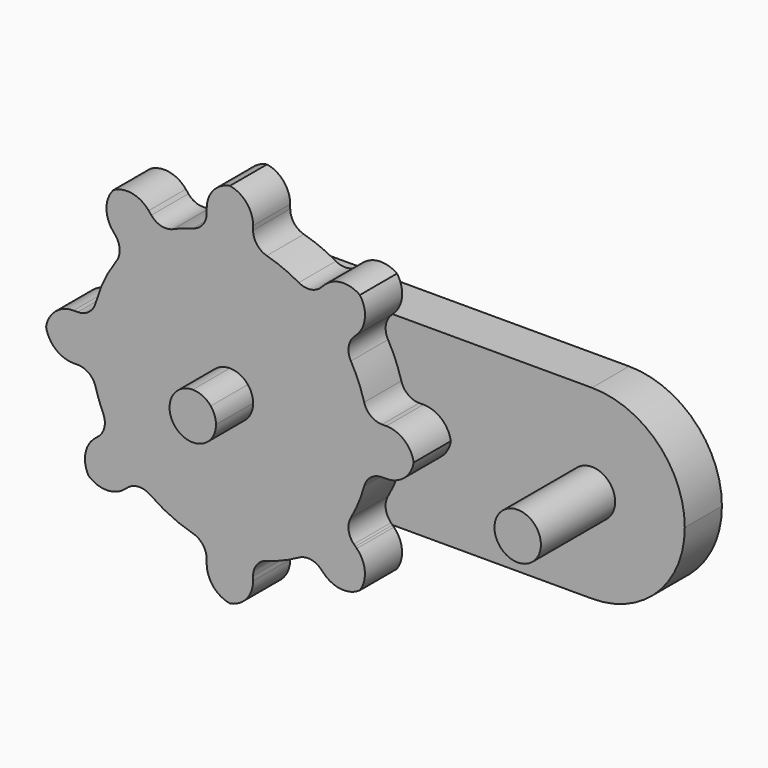
from build123d import *

# Parameters (mm, degrees)
F1_DEPTH    = 12.7
F3_DEPTH    = 25.4
F4_DEPTH    = 12.7
F5_T1_DEPTH = 50.8
F5_T3_DEPTH = 50.8226057065
F5_T5_DEPTH = 50.8231682345
F5_T7_DEPTH = 51.3109317266
F2_R        = 6.35
F6_DEPTH    = 25.4
F7_R        = 5.08


# Not quite as in the source:
# - a fillet or chamfer that OpenCascade refuses, or shapes differently, is made with other operations: its cross-section is extruded or revolved along the edge and cut away or added
# - a feature names something its author has since deleted; it is built from what else it names


with BuildPart() as f1:
    # F0 (on Front) → F1 (new body)
    with BuildSketch(Plane.XZ):
        with BuildLine():
            Line((50.8, 25.4), (0, 25.4))
            Line((0, 25.4), (-50.8, 25.4))
            ThreePointArc((-50.8, 25.4), (-32.8394877579, 17.9605122421), (-25.4, 0))
            ThreePointArc((-25.4, 0), (-32.8394877579, -17.9605122421), (-50.8, -25.4))
            Line((-50.8, -25.4), (50.8, -25.4))
            ThreePointArc((50.8, -25.4), (25.4, 0), (50.8, 25.4))
        make_face()
        with BuildLine():
            ThreePointArc((76.2, 0), (68.7605122421, 17.9605122421), (50.8, 25.4))
            Line((50.8, 25.4), (50.8, 0))
            Line((50.8, 0), (50.8, -25.4))
            ThreePointArc((50.8, -25.4), (68.7605122421, -17.9605122421), (76.2, 0))
        make_face()
        with BuildLine():
            Line((50.8, 0), (50.8, 25.4))
            ThreePointArc((50.8, 25.4), (25.4, 0), (50.8, -25.4))
            Line((50.8, -25.4), (50.8, 0))
        make_face()
        with BuildLine():
            ThreePointArc((-25.4, 0), (-32.8394877579, 17.9605122421), (-50.8, 25.4))
            Line((-50.8, 25.4), (-50.8, -25.4))
            ThreePointArc((-50.8, -25.4), (-32.8394877579, -17.9605122421), (-25.4, 0))
        make_face()
        with BuildLine():
            Line((-50.8, -25.4), (-50.8, 25.4))
            ThreePointArc((-50.8, 25.4), (-76.2, 0), (-50.8, -25.4))
        make_face()
    extrude(amount=F1_DEPTH)

    # F2 (on face) → F3 (join)
    with BuildSketch(Plane.XZ.offset(12.7)):
        with BuildLine():
            Line((-38.1, 0), (-38.1, 6.35))
            ThreePointArc((-38.1, 6.35), (-40.5300397853, 5.8666350357), (-42.5901280449, 4.4901280762))
            ThreePointArc((-42.5901280449, 4.4901280762), (-43.3184117467, 3.6181043161), (-43.8796412291, 2.6302561211))
            ThreePointArc((-43.8796412291, 2.6302561211), (-44.3057723857, 1.3456927946), (-44.45, 0))
            Line((-44.45, 0), (-38.1, 0))
        make_face()
        with BuildLine():
            ThreePointArc((-31.75, 0), (-32.1210860167, 2.1389454365), (-33.1909724663, 4.0278963086))
            ThreePointArc((-33.1909724663, 4.0278963086), (-35.384732201, 5.7401934445), (-38.1, 6.35))
            Line((-38.1, 6.35), (-38.1, 0))
            Line((-38.1, 0), (-31.75, 0))
        make_face()
        with BuildLine():
            ThreePointArc((-34.0440592308, -4.8858821595), (-32.3520558508, -2.6988216054), (-31.75, 0))
            Line((-31.75, 0), (-38.1, 0))
            Line((-38.1, 0), (-38.1, -6.35))
            ThreePointArc((-38.1, -6.35), (-35.9439447726, -5.9727653442), (-34.0440592308, -4.8858821595))
        make_face()
        with BuildLine():
            ThreePointArc((-42.1396767001, -4.8993379307), (-40.2461248962, -5.9763406805), (-38.1, -6.35))
            Line((-38.1, -6.35), (-38.1, 0))
            Line((-38.1, 0), (-44.45, 0))
            ThreePointArc((-44.45, 0), (-44.0789139833, -2.1389454365), (-43.0090275337, -4.0278963086))
            Line((-43.0090275337, -4.0278963086), (-42.1396767001, -4.8993379307))
        make_face()
    extrude(amount=F3_DEPTH)

    # F2 (on face) → F6 (join)
    with BuildSketch(Plane.XZ.offset(12.7)):
        with Locations((50.8, 0)):
            Circle(F2_R)
    extrude(amount=F6_DEPTH)


with BuildPart() as f4:
    # F2 (on face) → F4 (new body)
    with BuildSketch(Plane.XZ.offset(12.7)):
        with BuildLine():
            ThreePointArc((-44.45, 37.5671066227), (-38.1, 38.1), (-31.75, 37.5671066227))
            Line((-31.75, 37.5671066227), (-31.75, 50.4015624758))
            Line((-31.75, 50.4015624758), (-44.45, 50.4015624758))
            Line((-44.45, 50.4015624758), (-44.45, 37.5671066227))
        make_face()
        with BuildLine():
            Line((-21.6802561211, 25.4), (-16.0261722181, 31.054083903))
            ThreePointArc((-16.0261722181, 31.054083903), (-23.5197612269, 35.1998101887), (-31.75, 37.5671066227))
            Line((-31.75, 37.5671066227), (-31.75, 25.4))
            Line((-31.75, 25.4), (-21.6802561211, 25.4))
        make_face()
        Polygon((-40.7302561211, 6.35), (-37.6355270345, 9.4447290866), (-44.45, 17.7499169198), (-44.45, 6.35), align=None)
        Polygon((-44.45, 17.7499169198), (-44.45, 25.4), (-50.7269542822, 25.4), align=None)
        Polygon((-44.45, 2.6302561211), (-44.45, 6.35), (-51.5241743618, 6.35), (-46.6414025016, 0.3990867524), (-44.45, 2.1694751581), align=None)
        with BuildLine():
            Line((-75.3934442484, 6.35), (-51.5241743618, 6.35))
            Line((-51.5241743618, 6.35), (-64.0796310794, 21.6520529834))
            ThreePointArc((-64.0796310794, 21.6520529834), (-71.2237769542, 15.1006402158), (-75.3934442484, 6.35))
        make_face()
        Polygon((-35.0962770958, 6.35), (-31.75, 6.35), (-31.75, 15.3302561211), (-37.6355270345, 9.4447290866), align=None)
        with BuildLine():
            ThreePointArc((-62.9493278972, -28.8811513458), (-54.2929296323, -34.4876648952), (-44.45, -37.5671066227))
            Line((-44.45, -37.5671066227), (-44.45, -25.4))
            Line((-44.45, -25.4), (-50.8, -25.4))
            ThreePointArc((-50.8, -25.4), (-54.2464658379, -25.1650923548), (-57.6291835519, -24.4647144274))
            Line((-57.6291835519, -24.4647144274), (-62.9493278972, -28.8811513458))
        make_face()
        with BuildLine():
            Line((-46.6414025016, 0.3990867524), (-51.5241743618, 6.35))
            Line((-51.5241743618, 6.35), (-75.3934442484, 6.35))
            ThreePointArc((-75.3934442484, 6.35), (-75.9975542735, 3.2005091207), (-76.2, 1.847e-07))
            ThreePointArc((-76.2, 1.847e-07), (-75.9975542968, -3.2005089374), (-75.3934442484, -6.35))
            Line((-75.3934442484, -6.35), (-54.9954820613, -6.35))
            Line((-54.9954820613, -6.35), (-46.6414025016, 0.3990867524))
        make_face()
        with BuildLine():
            ThreePointArc((-31.75, -37.5671066227), (-23.5268945025, -35.2027640415), (-16.0387597828, -31.0630275421))
            Line((-16.0387597828, -31.0630275421), (-21.6882004226, -25.4))
            Line((-21.6882004226, -25.4), (-31.75, -25.4))
            Line((-31.75, -25.4), (-31.75, -37.5671066227))
        make_face()
        with BuildLine():
            Line((-3.7630761576, -25.4), (-7.0639290773, -22.0991470804))
            ThreePointArc((-7.0639290773, -22.0991470804), (-8.337137476, -23.786172756), (-9.7019366858, -25.4))
            Line((-9.7019366858, -25.4), (-3.7630761576, -25.4))
        make_face()
        with BuildLine():
            ThreePointArc((-16.0261722181, 31.054083903), (-12.7061993018, 28.4036069206), (-9.7019366858, 25.4))
            Line((-9.7019366858, 25.4), (-3.7197438789, 25.4))
            Line((-3.7197438789, 25.4), (2.0294146696, 31.1491585485))
            Line((2.0294146696, 31.1491585485), (-6.9508414515, 40.1294146696))
            Line((-6.9508414515, 40.1294146696), (-16.0261722181, 31.054083903))
        make_face()
        with BuildLine():
            Line((-21.6802561211, 25.4), (-9.7019366858, 25.4))
            ThreePointArc((-9.7019366858, 25.4), (-12.7061993018, 28.4036069206), (-16.0261722181, 31.054083903))
            Line((-16.0261722181, 31.054083903), (-21.6802561211, 25.4))
        make_face()
        Polygon((-44.45, -13.5242156334), (-38.479730006, -8.568086795), (-40.6924951019, -6.35), (-44.45, -6.35), align=None)
        with BuildLine():
            ThreePointArc((-75.6671066227, -6.35), (-73.9071383493, -13.0176358542), (-70.974125446, -19.2588129479))
            Line((-70.974125446, -19.2588129479), (-69.0293061757, -17.6876339953))
            ThreePointArc((-69.0293061757, -17.6876339953), (-72.9490964742, -12.4329210315), (-75.3934442484, -6.35))
            Line((-75.3934442484, -6.35), (-75.6671066227, -6.35))
        make_face()
        with BuildLine():
            Line((-57.6291835519, -24.4647144274), (-44.45, -13.5242156334))
            Line((-44.45, -13.5242156334), (-44.45, -6.35))
            Line((-44.45, -6.35), (-54.9954820613, -6.35))
            Line((-54.9954820613, -6.35), (-69.0293061757, -17.6876339953))
            ThreePointArc((-69.0293061757, -17.6876339953), (-63.7793752413, -21.8333647967), (-57.6291835519, -24.4647144274))
        make_face()
        with BuildLine():
            ThreePointArc((-9.7019366858, -25.4), (-8.337137476, -23.786172756), (-7.0639290773, -22.0991470804))
            Line((-7.0639290773, -22.0991470804), (-22.8130761576, -6.35))
            Line((-22.8130761576, -6.35), (-31.75, -6.35))
            Line((-31.75, -6.35), (-31.75, -15.3140017988))
            Line((-31.75, -15.3140017988), (-21.6882004226, -25.4))
            Line((-21.6882004226, -25.4), (-9.7019366858, -25.4))
        make_face()
        with BuildLine():
            ThreePointArc((-76.2, 1.847e-07), (-76.0665429105, 3.1861606087), (-75.6671066227, 6.35))
            Line((-75.6671066227, 6.35), (-88.5015624758, 6.35))
            Line((-88.5015624758, 6.35), (-88.5015624758, -6.35))
            Line((-88.5015624758, -6.35), (-75.6671066227, -6.35))
            ThreePointArc((-75.6671066227, -6.35), (-76.066542926, -3.1861604246), (-76.2, 1.847e-07))
        make_face()
        with BuildLine():
            ThreePointArc((-0.5328933773, 6.35), (-0.1334570818, 3.1861605167), (0, 0))
            ThreePointArc((0, 0), (-0.1334570818, -3.1861605167), (-0.5328933773, -6.35))
            Line((-0.5328933773, -6.35), (12.3015624758, -6.35))
            Line((12.3015624758, -6.35), (12.3015624758, 6.35))
            Line((12.3015624758, 6.35), (-0.5328933773, 6.35))
        make_face()
        with BuildLine():
            ThreePointArc((-0.5328933773, -6.35), (-0.1334570818, -3.1861605167), (0, 0))
            ThreePointArc((0, 0), (-0.1334570818, 3.1861605167), (-0.5328933773, 6.35))
            Line((-0.5328933773, 6.35), (-22.7697438789, 6.35))
            Line((-22.7697438789, 6.35), (-29.1414100183, -0.0216661394))
            Line((-29.1414100183, -0.0216661394), (-22.8130761576, -6.35))
            Line((-22.8130761576, -6.35), (-0.5328933773, -6.35))
        make_face()
        Polygon((-54.9954820613, -6.35), (-44.45, -6.35), (-44.45, -2.2717007737), (-46.6414025016, 0.3990867524), align=None)
        Polygon((-31.75, -25.4), (-31.75, -15.3140017988), (-38.479730006, -8.568086795), (-44.45, -13.5242156334), (-44.45, -25.4), align=None)
        Polygon((-29.1414100183, -0.0216661394), (-22.7697438789, 6.35), (-31.75, 6.35), (-31.75, 2.5869238424), align=None)
        with BuildLine():
            Line((-44.45, 25.4), (-44.45, 37.5671066227))
            ThreePointArc((-44.45, 37.5671066227), (-50.933672619, 35.8734838998), (-57.0203283861, 33.0700948557))
            Line((-57.0203283861, 33.0700948557), (-50.7269542822, 25.4))
            Line((-50.7269542822, 25.4), (-44.45, 25.4))
        make_face()
        with BuildLine():
            ThreePointArc((-70.974125446, -19.2588129479), (-67.3599831771, -24.4021184423), (-62.9493278972, -28.8811513458))
            Line((-62.9493278972, -28.8811513458), (-57.6291835519, -24.4647144274))
            ThreePointArc((-57.6291835519, -24.4647144274), (-63.7793752413, -21.8333647967), (-69.0293061757, -17.6876339953))
            Line((-69.0293061757, -17.6876339953), (-70.974125446, -19.2588129479))
        make_face()
        with BuildLine():
            Line((-50.7269542822, 25.4), (-57.0203283861, 33.0700948557))
            ThreePointArc((-57.0203283861, 33.0700948557), (-62.2673778517, 29.4541652025), (-66.8383834535, 25.0143022385))
            Line((-66.8383834535, 25.0143022385), (-64.0796310794, 21.6520529834))
            ThreePointArc((-64.0796310794, 21.6520529834), (-57.6991975701, 24.4450623417), (-50.8, 25.4))
            Line((-50.8, 25.4), (-50.7269542822, 25.4))
        make_face()
        Polygon((-37.6355270345, 9.4447290866), (-31.75, 15.3302561211), (-31.75, 25.4), (-44.45, 25.4), (-44.45, 17.7499169198), align=None)
        with BuildLine():
            ThreePointArc((-16.0387597828, -31.0630275421), (-12.7119556, -28.4087521997), (-9.7019366858, -25.4))
            Line((-9.7019366858, -25.4), (-21.6882004226, -25.4))
            Line((-21.6882004226, -25.4), (-16.0387597828, -31.0630275421))
        make_face()
        Polygon((-31.75, -6.35), (-22.8130761576, -6.35), (-29.1414100183, -0.0216661394), (-31.75, -2.6302561211), align=None)
        with BuildLine():
            ThreePointArc((-44.45, -37.5671066227), (-38.1, -38.1), (-31.75, -37.5671066227))
            Line((-31.75, -37.5671066227), (-31.75, -25.4))
            Line((-31.75, -25.4), (-44.45, -25.4))
            Line((-44.45, -25.4), (-44.45, -37.5671066227))
        make_face()
        with BuildLine():
            Line((-64.0796310794, 21.6520529834), (-66.8383834535, 25.0143022385))
            ThreePointArc((-66.8383834535, 25.0143022385), (-72.5411606668, 16.2916067939), (-75.6671066227, 6.35))
            Line((-75.6671066227, 6.35), (-75.3934442484, 6.35))
            ThreePointArc((-75.3934442484, 6.35), (-71.2237769542, 15.1006402158), (-64.0796310794, 21.6520529834))
        make_face()
        Polygon((-31.75, -15.3140017988), (-31.75, -6.35), (-35.8077702027, -6.35), (-38.479730006, -8.568086795), align=None)
        Polygon((-31.75, 15.3302561211), (-21.6802561211, 25.4), (-31.75, 25.4), align=None)
        Polygon((-31.75, -25.4), (-21.6882004226, -25.4), (-31.75, -15.3140017988), align=None)
        with BuildLine():
            ThreePointArc((-9.7019366858, 25.4), (-8.3274403588, 23.7740339953), (-7.045916097, 22.0738277819))
            Line((-7.045916097, 22.0738277819), (-3.7197438789, 25.4))
            Line((-3.7197438789, 25.4), (-9.7019366858, 25.4))
        make_face()
        with BuildLine():
            Line((-44.45, 6.35), (-44.45, 17.7499169198))
            Line((-44.45, 17.7499169198), (-50.7269542822, 25.4))
            Line((-50.7269542822, 25.4), (-50.8, 25.4))
            ThreePointArc((-50.8, 25.4), (-57.6991975701, 24.4450623417), (-64.0796310794, 21.6520529834))
            Line((-64.0796310794, 21.6520529834), (-51.5241743618, 6.35))
            Line((-51.5241743618, 6.35), (-44.45, 6.35))
        make_face()
        with BuildLine():
            ThreePointArc((-66.8383834535, 25.0143022385), (-62.2673778517, 29.4541652025), (-57.0203283861, 33.0700948557))
            Line((-57.0203283861, 33.0700948557), (-65.1614082843, 42.992094409))
            Line((-65.1614082843, 42.992094409), (-74.9794633518, 34.9363017918))
            Line((-74.9794633518, 34.9363017918), (-66.8383834535, 25.0143022385))
        make_face()
        with BuildLine():
            Line((-22.7697438789, 6.35), (-7.045916097, 22.0738277819))
            ThreePointArc((-7.045916097, 22.0738277819), (-8.3274403588, 23.7740339953), (-9.7019366858, 25.4))
            Line((-9.7019366858, 25.4), (-21.6802561211, 25.4))
            Line((-21.6802561211, 25.4), (-31.75, 15.3302561211))
            Line((-31.75, 15.3302561211), (-31.75, 6.35))
            Line((-31.75, 6.35), (-22.7697438789, 6.35))
        make_face()
        with BuildLine():
            Line((-31.75, 25.4), (-31.75, 37.5671066227))
            ThreePointArc((-31.75, 37.5671066227), (-38.1, 38.1), (-44.45, 37.5671066227))
            Line((-44.45, 37.5671066227), (-44.45, 25.4))
            Line((-44.45, 25.4), (-31.75, 25.4))
        make_face()
        with BuildLine():
            Line((-50.8, -25.4), (-44.45, -25.4))
            Line((-44.45, -25.4), (-44.45, -13.5242156334))
            Line((-44.45, -13.5242156334), (-57.6291835519, -24.4647144274))
            ThreePointArc((-57.6291835519, -24.4647144274), (-54.2464658379, -25.1650923548), (-50.8, -25.4))
        make_face()
        with BuildLine():
            Line((-3.7630761576, -25.4), (-9.7019366858, -25.4))
            ThreePointArc((-9.7019366858, -25.4), (-12.7119556, -28.4087521997), (-16.0387597828, -31.0630275421))
            Line((-16.0387597828, -31.0630275421), (-6.9752420892, -40.1483429919))
            Line((-6.9752420892, -40.1483429919), (2.0104715174, -31.1735476751))
            Line((2.0104715174, -31.1735476751), (-3.7630761576, -25.4))
        make_face()
        with BuildLine():
            Line((-69.0293061757, -17.6876339953), (-54.9954820613, -6.35))
            Line((-54.9954820613, -6.35), (-75.3934442484, -6.35))
            ThreePointArc((-75.3934442484, -6.35), (-72.9490964742, -12.4329210315), (-69.0293061757, -17.6876339953))
        make_face()
        with BuildLine():
            Line((-22.7697438789, 6.35), (-0.5328933773, 6.35))
            ThreePointArc((-0.5328933773, 6.35), (-2.9001898113, 14.5802387731), (-7.045916097, 22.0738277819))
            Line((-7.045916097, 22.0738277819), (-22.7697438789, 6.35))
        make_face()
        with BuildLine():
            ThreePointArc((-7.0639290773, -22.0991470804), (-2.9061383083, -14.5945914375), (-0.5328933773, -6.35))
            Line((-0.5328933773, -6.35), (-22.8130761576, -6.35))
            Line((-22.8130761576, -6.35), (-7.0639290773, -22.0991470804))
        make_face()
        with BuildLine():
            Line((-31.75, -50.4015624758), (-31.75, -37.5671066227))
            ThreePointArc((-31.75, -37.5671066227), (-38.1, -38.1), (-44.45, -37.5671066227))
            Line((-44.45, -37.5671066227), (-44.45, -50.4015624758))
            Line((-44.45, -50.4015624758), (-31.75, -50.4015624758))
        make_face()
        with BuildLine():
            Line((-72.8245466183, -37.0789139829), (-62.9493278972, -28.8811513458))
            ThreePointArc((-62.9493278972, -28.8811513458), (-67.3599831771, -24.4021184423), (-70.974125446, -19.2588129479))
            Line((-70.974125446, -19.2588129479), (-80.9364281568, -27.3071496639))
            Line((-80.9364281568, -27.3071496639), (-72.8245466183, -37.0789139829))
        make_face()
        with BuildLine():
            Line((-44.45, -6.35), (-40.6924951019, -6.35))
            Line((-40.6924951019, -6.35), (-42.1396767001, -4.8993379307))
            ThreePointArc((-42.1396767001, -4.8993379307), (-42.5955177112, -4.4847319328), (-43.0090275337, -4.0278963086))
            Line((-43.0090275337, -4.0278963086), (-44.45, -2.2717007737))
            Line((-44.45, -2.2717007737), (-44.45, -6.35))
        make_face()
        with BuildLine():
            Line((-75.3934442484, 6.35), (-75.6671066227, 6.35))
            ThreePointArc((-75.6671066227, 6.35), (-76.0665429105, 3.1861606087), (-76.2, 1.847e-07))
            ThreePointArc((-76.2, 1.847e-07), (-75.9975542735, 3.2005091207), (-75.3934442484, 6.35))
        make_face()
        with BuildLine():
            Line((-35.8077702027, -6.35), (-31.75, -6.35))
            Line((-31.75, -6.35), (-31.75, -2.6302561211))
            Line((-31.75, -2.6302561211), (-31.75, 0))
            ThreePointArc((-31.75, 0), (-32.3520558508, -2.6988216054), (-34.0440592308, -4.8858821595))
            Line((-34.0440592308, -4.8858821595), (-35.8077702027, -6.35))
        make_face()
        Polygon((-31.75, 2.5869238424), (-31.75, 6.35), (-35.0962770958, 6.35), (-33.1909724663, 4.0278963086), align=None)
        with BuildLine():
            ThreePointArc((-43.8796412291, 2.6302561211), (-43.3184117467, 3.6181043161), (-42.5901280449, 4.4901280762))
            Line((-42.5901280449, 4.4901280762), (-44.45, 2.6302561211))
            Line((-44.45, 2.6302561211), (-44.45, 2.1694751581))
            Line((-44.45, 2.1694751581), (-43.8796412291, 2.6302561211))
        make_face()
        Polygon((-42.5901280449, 4.4901280762), (-40.7302561211, 6.35), (-44.45, 6.35), (-44.45, 2.6302561211), align=None)
        with BuildLine():
            Line((-33.1909724663, 4.0278963086), (-35.0962770958, 6.35))
            Line((-35.0962770958, 6.35), (-38.1, 6.35))
            ThreePointArc((-38.1, 6.35), (-35.384732201, 5.7401934445), (-33.1909724663, 4.0278963086))
        make_face()
        with BuildLine():
            ThreePointArc((-76.2, 1.847e-07), (-76.066542926, -3.1861604246), (-75.6671066227, -6.35))
            Line((-75.6671066227, -6.35), (-75.3934442484, -6.35))
            ThreePointArc((-75.3934442484, -6.35), (-75.9975542968, -3.2005089374), (-76.2, 1.847e-07))
        make_face()
        Polygon((-38.1, 6.35), (-35.0962770958, 6.35), (-37.6355270345, 9.4447290866), (-40.7302561211, 6.35), align=None)
        Polygon((-31.75, -2.6302561211), (-29.1414100183, -0.0216661394), (-31.75, 2.5869238424), (-31.75, 2.2717007737), (-31.75, 0), align=None)
        Polygon((-31.75, 2.2717007737), (-31.75, 2.5869238424), (-33.1909724663, 4.0278963086), align=None)
        with BuildLine():
            ThreePointArc((-42.5901280449, 4.4901280762), (-40.5300397853, 5.8666350357), (-38.1, 6.35))
            Line((-38.1, 6.35), (-40.7302561211, 6.35))
            Line((-40.7302561211, 6.35), (-42.5901280449, 4.4901280762))
        make_face()
        with BuildLine():
            Line((-40.6924951019, -6.35), (-38.1, -6.35))
            ThreePointArc((-38.1, -6.35), (-40.2461248962, -5.9763406805), (-42.1396767001, -4.8993379307))
            Line((-42.1396767001, -4.8993379307), (-40.6924951019, -6.35))
        make_face()
        with BuildLine():
            Line((-38.1, -6.35), (-35.8077702027, -6.35))
            Line((-35.8077702027, -6.35), (-34.0440592308, -4.8858821595))
            ThreePointArc((-34.0440592308, -4.8858821595), (-35.9439447726, -5.9727653442), (-38.1, -6.35))
        make_face()
        with BuildLine():
            ThreePointArc((-43.0090275337, -4.0278963086), (-44.0789139833, -2.1389454365), (-44.45, 0))
            Line((-44.45, 0), (-44.45, -2.2717007737))
            Line((-44.45, -2.2717007737), (-43.0090275337, -4.0278963086))
        make_face()
        with BuildLine():
            Line((-31.75, 0), (-31.75, 2.2717007737))
            Line((-31.75, 2.2717007737), (-33.1909724663, 4.0278963086))
            ThreePointArc((-33.1909724663, 4.0278963086), (-32.1210860167, 2.1389454365), (-31.75, 0))
        make_face()
        with BuildLine():
            ThreePointArc((-43.0090275337, -4.0278963086), (-42.5955177112, -4.4847319328), (-42.1396767001, -4.8993379307))
            Line((-42.1396767001, -4.8993379307), (-43.0090275337, -4.0278963086))
        make_face()
        Polygon((-38.479730006, -8.568086795), (-35.8077702027, -6.35), (-38.1, -6.35), (-40.6924951019, -6.35), align=None)
        Polygon((-44.45, -2.2717007737), (-44.45, 0), (-44.45, 2.1694751581), (-46.6414025016, 0.3990867524), align=None)
        with BuildLine():
            ThreePointArc((-44.45, 0), (-44.3057723857, 1.3456927946), (-43.8796412291, 2.6302561211))
            Line((-43.8796412291, 2.6302561211), (-44.45, 2.1694751581))
            Line((-44.45, 2.1694751581), (-44.45, 0))
        make_face()
    extrude(amount=F4_DEPTH)

    # F5: fillet of radius 7.62 on 16 edges, made by hand

    # F5_s2 → F5_t1 (cut)
    with BuildSketch(Plane.XZ.offset(-6.35)):
        with BuildLine():
            ThreePointArc((-60.3279327139, 37.1012613685), (-65.4711011172, 39.8510171404), (-71.0522413248, 38.1586188387))
            Line((-71.0522413248, 38.1586188387), (-65.1614082843, 42.992094409))
            Line((-65.1614082843, 42.992094409), (-60.3279327139, 37.1012613685))
        make_face()
        with BuildLine():
            ThreePointArc((-69.0886303113, 39.7697773621), (-71.8383860832, 34.6266089589), (-70.1459877814, 29.0454687513))
            Line((-70.1459877814, 29.0454687513), (-74.9794633518, 34.9363017918))
            Line((-74.9794633518, 34.9363017918), (-69.0886303113, 39.7697773621))
        make_face()
        with BuildLine():
            ThreePointArc((-36.83, 50.4015624758), (-42.2181536726, 48.1697161484), (-44.45, 42.7815624758))
            Line((-44.45, 42.7815624758), (-44.45, 50.4015624758))
            Line((-44.45, 50.4015624758), (-36.83, 50.4015624758))
        make_face()
        with BuildLine():
            ThreePointArc((-31.75, 42.7815624758), (-33.9818463274, 48.1697161484), (-39.37, 50.4015624758))
            Line((-39.37, 50.4015624758), (-31.75, 50.4015624758))
            Line((-31.75, 50.4015624758), (-31.75, 42.7815624758))
        make_face()
        with BuildLine():
            ThreePointArc((-1.5626877789, 34.7412609969), (-6.9508414515, 36.9731073243), (-12.3389951242, 34.7412609969))
            Line((-12.3389951242, 34.7412609969), (-6.9508414515, 40.1294146696))
            Line((-6.9508414515, 40.1294146696), (-1.5626877789, 34.7412609969))
        make_face()
        with BuildLine():
            ThreePointArc((-3.3587390031, 25.7610048758), (-1.1268926757, 31.1491585485), (-3.3587390031, 36.5373122211))
            Line((-3.3587390031, 36.5373122211), (2.0294146696, 31.1491585485))
            Line((2.0294146696, 31.1491585485), (-3.3587390031, 25.7610048758))
        make_face()
        with BuildLine():
            ThreePointArc((12.3015624758, -1.27), (10.0697161484, 4.1181536726), (4.6815624758, 6.35))
            Line((4.6815624758, 6.35), (12.3015624758, 6.35))
            Line((12.3015624758, 6.35), (12.3015624758, -1.27))
        make_face()
        with BuildLine():
            ThreePointArc((4.6815624758, -6.35), (10.0697161484, -4.1181536726), (12.3015624758, 1.27))
            Line((12.3015624758, 1.27), (12.3015624758, -6.35))
            Line((12.3015624758, -6.35), (4.6815624758, -6.35))
        make_face()
        with BuildLine():
            ThreePointArc((-39.37, -50.4015624758), (-33.9818463274, -48.1697161484), (-31.75, -42.7815624758))
            Line((-31.75, -42.7815624758), (-31.75, -50.4015624758))
            Line((-31.75, -50.4015624758), (-39.37, -50.4015624758))
        make_face()
        with BuildLine():
            ThreePointArc((-44.45, -42.7815624758), (-42.2181536726, -48.1697161484), (-36.83, -50.4015624758))
            Line((-36.83, -50.4015624758), (-44.45, -50.4015624758))
            Line((-44.45, -50.4015624758), (-44.45, -42.7815624758))
        make_face()
        with BuildLine():
            ThreePointArc((-77.6916755414, -31.2158553915), (-72.5328455721, -33.9361148233), (-66.961488027, -32.2117850598))
            Line((-66.961488027, -32.2117850598), (-72.8245466183, -37.0789139829))
            Line((-72.8245466183, -37.0789139829), (-77.6916755414, -31.2158553915))
        make_face()
        with BuildLine():
            ThreePointArc((-88.5015624758, 1.27), (-86.2697161484, -4.1181536726), (-80.8815624758, -6.35))
            Line((-80.8815624758, -6.35), (-88.5015624758, -6.35))
            Line((-88.5015624758, -6.35), (-88.5015624758, 1.27))
        make_face()
        with BuildLine():
            ThreePointArc((-80.8815624758, 6.35), (-86.2697161484, 4.1181536726), (-88.5015624758, -1.27))
            Line((-88.5015624758, -1.27), (-88.5015624758, 6.35))
            Line((-88.5015624758, 6.35), (-80.8815624758, 6.35))
        make_face()
    extrude(amount=F5_T1_DEPTH, mode=Mode.SUBTRACT)

    # F5_s4 → F5_t3 (cut)
    with BuildSketch(Plane.XZ.offset(-6.3613028533)):
        with BuildLine():
            ThreePointArc((-12.3601134962, -34.7505209715), (-6.9723843804, -36.9888395353), (-1.5806150527, -34.7602708162))
            Line((-1.5806150527, -34.7602708162), (-6.9752420892, -40.1483429919))
            Line((-6.9752420892, -40.1483429919), (-12.3601134962, -34.7505209715))
        make_face()
    extrude(amount=F5_T3_DEPTH, mode=Mode.SUBTRACT)

    # F5_s6 → F5_t5 (cut)
    with BuildSketch(Plane.XZ.offset(-6.3615841172)):
        with BuildLine():
            ThreePointArc((-3.3842351209, -36.5616993559), (-1.149112663, -31.1725873111), (-3.3809586384, -25.7821175193))
            Line((-3.3809586384, -25.7821175193), (2.0104715174, -31.1735476751))
            Line((2.0104715174, -31.1735476751), (-3.3842351209, -36.5616993559))
        make_face()
    extrude(amount=F5_T5_DEPTH, mode=Mode.SUBTRACT)

    # F5_s8 → F5_t7 (cut)
    with BuildSketch(Plane.XZ.offset(-6.6054658633)):
        with BuildLine():
            ThreePointArc((-74.9295700645, -22.4543342119), (-77.7235007403, -27.6269570591), (-76.0040296646, -33.2488335217))
            Line((-76.0040296646, -33.2488335217), (-80.9364281568, -27.3071496639))
            Line((-80.9364281568, -27.3071496639), (-74.9295700645, -22.4543342119))
        make_face()
    extrude(amount=F5_T7_DEPTH, mode=Mode.SUBTRACT)

    # F7
    f7_edges = [f4.edges().sort_by_distance(p)[0] for p in [
        (-31.75, -19.05, 37.567107),
        (-16.026172, -19.05, 31.054084),
        (-44.45, -19.05, 37.567107),
        (-57.020328, -19.05, 33.070095),
        (-75.667107, -19.05, 6.35),
        (-66.838383, -19.05, 25.014302),
        (-75.667107, -19.05, -6.35),
        (-70.974125, -19.05, -19.258813),
        (-62.949328, -19.05, -28.881151),
        (-44.45, -19.05, -37.567107),
        (-31.75, -19.05, -37.567107),
        (-16.03876, -19.05, -31.063028),
        (-7.063929, -19.05, -22.099147),
        (-7.045916, -19.05, 22.073828),
        (-0.532893, -19.05, 6.35),
        (-0.532893, -19.05, -6.35),
    ]]
    fillet(f7_edges, radius=F7_R)


solid = Compound([f1.part, f4.part])
